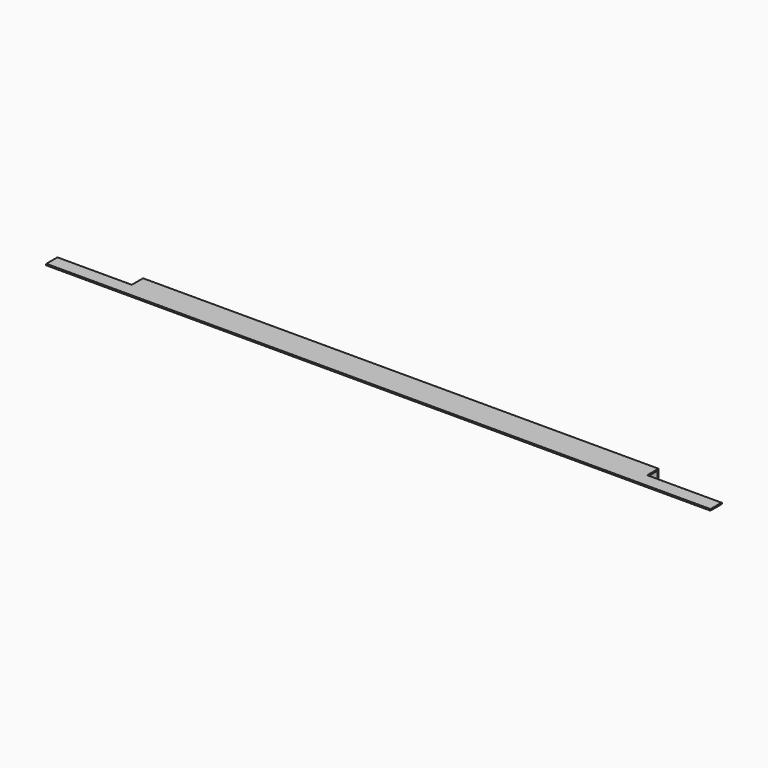
from build123d import *

# Parameters (mm, degrees)
F0_W           = 50.1573085785
F0_H           = 16.5988057852
F1_DEPTH       = 38
F2_DEPTH       = 2
F3_DEPTH       = 894
F4_W           = 19
F4_H           = 2
F5_DEPTH       = 100
F6_W           = 19
F6_H           = 2
F7_DEPTH       = 100
F8_W           = 694
F8_H           = 9.5
F9_DEPTH       = 10
F10_DEPTH      = 7.5
F11_T1_DEPTH   = 21.5048292256
F11_T3_DEPTH   = 101.2524146128
F11_T5_DEPTH   = 17
F11_T7_DEPTH   = 10.9980686292
F11_T9_DEPTH   = 11.2524146128
F11_T11_DEPTH  = 2.7514489274
F11_T13_DEPTH  = 692.9980686292
F11_T15_DEPTH  = 101.2524146128
F11_T17_DEPTH  = 18.4990343146
F11_S21_W      = 0.5515022539
F11_S21_H      = 0.5515022539
F11_T22_DEPTH  = 0.551502254
F11_S27_W      = 0.5515022539
F11_S27_H      = 0.5515022539
F11_T28_DEPTH  = 0.551502254
F11_S33_W      = 0.5515022539
F11_S33_H      = 0.5515022539
F11_T34_DEPTH  = 0.551502254
F11_S39_W      = 0.5515022539
F11_S39_H      = 0.5515022539
F11_T40_DEPTH  = 0.551502254
F11_T47_DEPTH  = 101.2524146128
F11_T51_DEPTH  = 18.2524146128
F11_T58_DEPTH  = 18.2524146128
F11_T62_DEPTH  = 11.2524146128
F11_T69_DEPTH  = 19.7514489274
F11_T73_DEPTH  = 101.2524146128
F11_T80_DEPTH  = 18.2524146128
F11_T84_DEPTH  = 11.2524146128
F11_T91_DEPTH  = 18.2524146128
F11_T95_DEPTH  = 101.2524146128
F11_T102_DEPTH = 19.7514489274
F11_T106_DEPTH = 101.2524146128


# Not quite as in the source:
# - a fillet or chamfer that OpenCascade refuses, or shapes differently, is made with other operations: its cross-section is extruded or revolved along the edge and cut away or added
# - a feature names something its author has since deleted; it is built from what else it names


with BuildPart() as f1:
    # F0 (on Front) → F1 (new body)
    with BuildSketch(Plane.XZ):
        with Locations((-25.0786542892, 8.2994028926)):
            Rectangle(F0_W, F0_H)
    extrude(amount=-F1_DEPTH)

    # F2 (intersect): a face of the model
    f2_faces = [f1.faces().sort_by_distance(p)[0] for p in [
        (-25.0786542892, 19, 0),
    ]]
    extrude(f2_faces, amount=-F2_DEPTH, mode=Mode.INTERSECT)

    # F3 (add): a face of the model
    f3_faces = [f1.faces().sort_by_distance(p)[0] for p in [
        (0, 19, 1),
    ]]
    extrude(f3_faces, amount=-F3_DEPTH)

    # F4 (on face) → F5 (cut)
    with BuildSketch(Plane.YZ):
        with Locations((28.5, 1)):
            Rectangle(F4_W, F4_H)
    extrude(amount=-F5_DEPTH, mode=Mode.SUBTRACT)

    # F6 (on face) → F7 (cut)
    with BuildSketch(Plane(origin=(-894, 0, 0), x_dir=(0, -1, 0), z_dir=(-1, 0, 0))):
        with Locations((-28.5, 1)):
            Rectangle(F6_W, F6_H)
    extrude(amount=-F7_DEPTH, mode=Mode.SUBTRACT)

    # F8 (on face) → F9 (join)
    with BuildSketch(Plane(origin=(0, 0, 0), x_dir=(1, 0, 0), z_dir=(0, 0, -1))):
        with Locations((-447, -33.25)):
            Rectangle(F8_W, F8_H)
    extrude(amount=F9_DEPTH)

    # F10 (cut): a face of the model
    f10_faces = [f1.faces().sort_by_distance(p)[0] for p in [
        (-447, 28.5, -5),
    ]]
    extrude(f10_faces, amount=-F10_DEPTH, mode=Mode.SUBTRACT)

    # F11: fillet of radius 0.5 on 21 edges, made by hand

    # F11_s2 → F11_t1 (cut)
    with BuildSketch(Plane.XZ.offset(-20.2524146128)):
        with BuildLine():
            ThreePointArc((-893.4990343146, -0.0004), (-893.8535533906, 0.1464466094), (-894.0004, 0.5009656854))
            Line((-894.0004, 0.5009656854), (-894.0505365685, 0.5009656854))
            ThreePointArc((-894.0505365685, 0.5009656854), (-894.0501365685, 0.2504828427), (-894.0501365685, 0))
            Line((-894.0501365685, 0), (-894, -0.0501365685))
            ThreePointArc((-894, -0.0501365685), (-893.7495171573, -0.0501365685), (-893.4990343146, -0.0505365685))
            Line((-893.4990343146, -0.0505365685), (-893.4990343146, -0.0004))
        make_face()
        with BuildLine():
            ThreePointArc((0.0004, 0.5009656854), (-0.1464466094, 0.1464466094), (-0.5009656854, -0.0004))
            Line((-0.5009656854, -0.0004), (-0.5009656854, -0.0505365685))
            ThreePointArc((-0.5009656854, -0.0505365685), (-0.2504828427, -0.0501365685), (0, -0.0501365685))
            Line((0, -0.0501365685), (0.0501365685, 0))
            ThreePointArc((0.0501365685, 0), (0.0501365685, 0.2504828427), (0.0505365685, 0.5009656854))
            Line((0.0505365685, 0.5009656854), (0.0004, 0.5009656854))
        make_face()
        with BuildLine():
            ThreePointArc((0.0004, 1.4990343146), (-0.1464466094, 1.8535533906), (-0.5009656854, 2.0004))
            Line((-0.5009656854, 2.0004), (-0.5009656854, 2.0505365685))
            ThreePointArc((-0.5009656854, 2.0505365685), (-0.2504828427, 2.0501365685), (0, 2.0501365685))
            Line((0, 2.0501365685), (0.0501365685, 2))
            ThreePointArc((0.0501365685, 2), (0.0501365685, 1.7495171573), (0.0505365685, 1.4990343146))
            Line((0.0505365685, 1.4990343146), (0.0004, 1.4990343146))
        make_face()
        with BuildLine():
            ThreePointArc((-894.0004, 1.4990343146), (-893.8535533906, 1.8535533906), (-893.4990343146, 2.0004))
            Line((-893.4990343146, 2.0004), (-893.4990343146, 2.0505365685))
            ThreePointArc((-893.4990343146, 2.0505365685), (-893.7495171573, 2.0501365685), (-894, 2.0501365685))
            Line((-894, 2.0501365685), (-894.0501365685, 2))
            ThreePointArc((-894.0501365685, 2), (-894.0501365685, 1.7495171573), (-894.0505365685, 1.4990343146))
            Line((-894.0505365685, 1.4990343146), (-894.0004, 1.4990343146))
        make_face()
    extrude(amount=F11_T1_DEPTH, mode=Mode.SUBTRACT)

    # F11_s4 → F11_t3 (cut)
    with BuildSketch(Plane.YZ.offset(-895.2524146128)):
        with BuildLine():
            ThreePointArc((18.4990343146, -0.0004), (18.8535533906, 0.1464466094), (19.0004, 0.5009656854))
            Line((19.0004, 0.5009656854), (19.0505365685, 0.5009656854))
            ThreePointArc((19.0505365685, 0.5009656854), (19.0501365685, 0.2504828427), (19.0501365685, 0))
            Line((19.0501365685, 0), (19, -0.0501365685))
            ThreePointArc((19, -0.0501365685), (18.7495171573, -0.0501365685), (18.4990343146, -0.0505365685))
            Line((18.4990343146, -0.0505365685), (18.4990343146, -0.0004))
        make_face()
        with BuildLine():
            ThreePointArc((19.0004, 1.4990343146), (18.8535533906, 1.8535533906), (18.4990343146, 2.0004))
            Line((18.4990343146, 2.0004), (18.4990343146, 2.0505365685))
            ThreePointArc((18.4990343146, 2.0505365685), (18.7495171573, 2.0501365685), (19, 2.0501365685))
            Line((19, 2.0501365685), (19.0501365685, 2))
            ThreePointArc((19.0501365685, 2), (19.0501365685, 1.7495171573), (19.0505365685, 1.4990343146))
            Line((19.0505365685, 1.4990343146), (19.0004, 1.4990343146))
        make_face()
    extrude(amount=F11_T3_DEPTH, mode=Mode.SUBTRACT)

    # F11_s6 → F11_t5 (cut)
    with BuildSketch(Plane.XZ.offset(-36)):
        with BuildLine():
            ThreePointArc((-793.4990343146, -0.0004), (-793.8535533906, 0.1464466094), (-794.0004, 0.5009656854))
            Line((-794.0004, 0.5009656854), (-794.0505365685, 0.5009656854))
            ThreePointArc((-794.0505365685, 0.5009656854), (-794.0501365685, 0.2504828427), (-794.0501365685, 0))
            Line((-794.0501365685, 0), (-794, -0.0501365685))
            ThreePointArc((-794, -0.0501365685), (-793.7495171573, -0.0501365685), (-793.4990343146, -0.0505365685))
            Line((-793.4990343146, -0.0505365685), (-793.4990343146, -0.0004))
        make_face()
        with BuildLine():
            ThreePointArc((-100.5009656854, -0.0004), (-100.1464466094, 0.1464466094), (-99.9996, 0.5009656854))
            Line((-99.9996, 0.5009656854), (-99.9494634315, 0.5009656854))
            ThreePointArc((-99.9494634315, 0.5009656854), (-99.9498634315, 0.2504828427), (-99.9498634315, 0))
            Line((-99.9498634315, 0), (-100, -0.0501365685))
            ThreePointArc((-100, -0.0501365685), (-100.2504828427, -0.0501365685), (-100.5009656854, -0.0505365685))
            Line((-100.5009656854, -0.0505365685), (-100.5009656854, -0.0004))
        make_face()
    extrude(amount=F11_T5_DEPTH, mode=Mode.SUBTRACT)

    # F11_s8 → F11_t7 (cut)
    with BuildSketch(Plane.XY.offset(-9.4990343146)):
        with BuildLine():
            ThreePointArc((-793.4990343146, 38.0004), (-793.8535533906, 37.8535533906), (-794.0004, 37.4990343146))
            Line((-794.0004, 37.4990343146), (-794.0505365685, 37.4990343146))
            ThreePointArc((-794.0505365685, 37.4990343146), (-794.0501365685, 37.7495171573), (-794.0501365685, 38))
            Line((-794.0501365685, 38), (-794, 38.0501365685))
            ThreePointArc((-794, 38.0501365685), (-793.7495171573, 38.0501365685), (-793.4990343146, 38.0505365685))
            Line((-793.4990343146, 38.0505365685), (-793.4990343146, 38.0004))
        make_face()
        with BuildLine():
            ThreePointArc((-99.9996, 37.4990343146), (-100.1464466094, 37.8535533906), (-100.5009656854, 38.0004))
            Line((-100.5009656854, 38.0004), (-100.5009656854, 38.0505365685))
            ThreePointArc((-100.5009656854, 38.0505365685), (-100.2504828427, 38.0501365685), (-100, 38.0501365685))
            Line((-100, 38.0501365685), (-99.9498634315, 38))
            ThreePointArc((-99.9498634315, 38), (-99.9498634315, 37.7495171573), (-99.9494634315, 37.4990343146))
            Line((-99.9494634315, 37.4990343146), (-99.9996, 37.4990343146))
        make_face()
    extrude(amount=F11_T7_DEPTH, mode=Mode.SUBTRACT)

    # F11_s10 → F11_t9 (cut)
    with BuildSketch(Plane.XY.offset(-11.2524146128)):
        with BuildLine():
            ThreePointArc((-793.4990343146, 35.9996), (-793.8535533906, 36.1464466094), (-794.0004, 36.5009656854))
            Line((-794.0004, 36.5009656854), (-794.0505365685, 36.5009656854))
            ThreePointArc((-794.0505365685, 36.5009656854), (-794.0501365685, 36.2504828427), (-794.0501365685, 36))
            Line((-794.0501365685, 36), (-794, 35.9498634315))
            ThreePointArc((-794, 35.9498634315), (-793.7495171573, 35.9498634315), (-793.4990343146, 35.9494634315))
            Line((-793.4990343146, 35.9494634315), (-793.4990343146, 35.9996))
        make_face()
        with BuildLine():
            ThreePointArc((-99.9996, 36.5009656854), (-100.1464466094, 36.1464466094), (-100.5009656854, 35.9996))
            Line((-100.5009656854, 35.9996), (-100.5009656854, 35.9494634315))
            ThreePointArc((-100.5009656854, 35.9494634315), (-100.2504828427, 35.9498634315), (-100, 35.9498634315))
            Line((-100, 35.9498634315), (-99.9498634315, 36))
            ThreePointArc((-99.9498634315, 36), (-99.9498634315, 36.2504828427), (-99.9494634315, 36.5009656854))
            Line((-99.9494634315, 36.5009656854), (-99.9996, 36.5009656854))
        make_face()
    extrude(amount=F11_T9_DEPTH, mode=Mode.SUBTRACT)

    # F11_s12 → F11_t11 (cut)
    with BuildSketch(Plane.XZ.offset(-37.4990343146)):
        with BuildLine():
            ThreePointArc((-793.4990343146, -10.0004), (-793.8535533906, -9.8535533906), (-794.0004, -9.4990343146))
            Line((-794.0004, -9.4990343146), (-794.0505365685, -9.4990343146))
            ThreePointArc((-794.0505365685, -9.4990343146), (-794.0501365685, -9.7495171573), (-794.0501365685, -10))
            Line((-794.0501365685, -10), (-794, -10.0501365685))
            ThreePointArc((-794, -10.0501365685), (-793.7495171573, -10.0501365685), (-793.4990343146, -10.0505365685))
            Line((-793.4990343146, -10.0505365685), (-793.4990343146, -10.0004))
        make_face()
        with BuildLine():
            ThreePointArc((-99.9996, -9.4990343146), (-100.1464466094, -9.8535533906), (-100.5009656854, -10.0004))
            Line((-100.5009656854, -10.0004), (-100.5009656854, -10.0505365685))
            ThreePointArc((-100.5009656854, -10.0505365685), (-100.2504828427, -10.0501365685), (-100, -10.0501365685))
            Line((-100, -10.0501365685), (-99.9498634315, -10))
            ThreePointArc((-99.9498634315, -10), (-99.9498634315, -9.7495171573), (-99.9494634315, -9.4990343146))
            Line((-99.9494634315, -9.4990343146), (-99.9996, -9.4990343146))
        make_face()
    extrude(amount=F11_T11_DEPTH, mode=Mode.SUBTRACT)

    # F11_s14 → F11_t13 (cut)
    with BuildSketch(Plane.YZ.offset(-793.4990343146)):
        with BuildLine():
            ThreePointArc((37.4990343146, -10.0004), (37.8535533906, -9.8535533906), (38.0004, -9.4990343146))
            Line((38.0004, -9.4990343146), (38.0505365685, -9.4990343146))
            ThreePointArc((38.0505365685, -9.4990343146), (38.0501365685, -9.7495171573), (38.0501365685, -10))
            Line((38.0501365685, -10), (38, -10.0501365685))
            ThreePointArc((38, -10.0501365685), (37.7495171573, -10.0501365685), (37.4990343146, -10.0505365685))
            Line((37.4990343146, -10.0505365685), (37.4990343146, -10.0004))
        make_face()
        with BuildLine():
            ThreePointArc((38.0004, 1.4990343146), (37.8535533906, 1.8535533906), (37.4990343146, 2.0004))
            Line((37.4990343146, 2.0004), (37.4990343146, 2.0505365685))
            ThreePointArc((37.4990343146, 2.0505365685), (37.7495171573, 2.0501365685), (38, 2.0501365685))
            Line((38, 2.0501365685), (38.0501365685, 2))
            ThreePointArc((38.0501365685, 2), (38.0501365685, 1.7495171573), (38.0505365685, 1.4990343146))
            Line((38.0505365685, 1.4990343146), (38.0004, 1.4990343146))
        make_face()
    extrude(amount=F11_T13_DEPTH, mode=Mode.SUBTRACT)

    # F11_s16 → F11_t15 (cut)
    with BuildSketch(Plane.YZ.offset(-100)):
        with BuildLine():
            ThreePointArc((19.0004, 1.4990343146), (18.8535533906, 1.8535533906), (18.4990343146, 2.0004))
            Line((18.4990343146, 2.0004), (18.4990343146, 2.0505365685))
            ThreePointArc((18.4990343146, 2.0505365685), (18.7495171573, 2.0501365685), (19, 2.0501365685))
            Line((19, 2.0501365685), (19.0501365685, 2))
            ThreePointArc((19.0501365685, 2), (19.0501365685, 1.7495171573), (19.0505365685, 1.4990343146))
            Line((19.0505365685, 1.4990343146), (19.0004, 1.4990343146))
        make_face()
        with BuildLine():
            ThreePointArc((18.4990343146, -0.0004), (18.8535533906, 0.1464466094), (19.0004, 0.5009656854))
            Line((19.0004, 0.5009656854), (19.0505365685, 0.5009656854))
            ThreePointArc((19.0505365685, 0.5009656854), (19.0501365685, 0.2504828427), (19.0501365685, 0))
            Line((19.0501365685, 0), (19, -0.0501365685))
            ThreePointArc((19, -0.0501365685), (18.7495171573, -0.0501365685), (18.4990343146, -0.0505365685))
            Line((18.4990343146, -0.0505365685), (18.4990343146, -0.0004))
        make_face()
    extrude(amount=F11_T15_DEPTH, mode=Mode.SUBTRACT)

    # F11_s18 → F11_t17 (cut)
    with BuildSketch(Plane.XZ.offset(-37.4990343146)):
        with BuildLine():
            ThreePointArc((-99.9996, 1.4990343146), (-100.1464466094, 1.8535533906), (-100.5009656854, 2.0004))
            Line((-100.5009656854, 2.0004), (-100.5009656854, 2.0505365685))
            ThreePointArc((-100.5009656854, 2.0505365685), (-100.2504828427, 2.0501365685), (-100, 2.0501365685))
            Line((-100, 2.0501365685), (-99.9498634315, 2))
            ThreePointArc((-99.9498634315, 2), (-99.9498634315, 1.7495171573), (-99.9494634315, 1.4990343146))
            Line((-99.9494634315, 1.4990343146), (-99.9996, 1.4990343146))
        make_face()
        with BuildLine():
            ThreePointArc((-794.0004, 1.4990343146), (-793.8535533906, 1.8535533906), (-793.4990343146, 2.0004))
            Line((-793.4990343146, 2.0004), (-793.4990343146, 2.0505365685))
            ThreePointArc((-793.4990343146, 2.0505365685), (-793.7495171573, 2.0501365685), (-794, 2.0501365685))
            Line((-794, 2.0501365685), (-794.0501365685, 2))
            ThreePointArc((-794.0501365685, 2), (-794.0501365685, 1.7495171573), (-794.0505365685, 1.4990343146))
            Line((-794.0505365685, 1.4990343146), (-794.0004, 1.4990343146))
        make_face()
    extrude(amount=F11_T17_DEPTH, mode=Mode.SUBTRACT)


with BuildPart() as f11_tool20:
    # F11_s21 → F11_t22 (new body)
    with BuildSketch(Plane.XY.offset(-9.4990343146)):
        with Locations((-793.7747854415, 37.7747854416)):
            Rectangle(F11_S21_W, F11_S21_H)
    extrude(amount=-F11_T22_DEPTH)

    # F11_s23 → F11_t24 (revolve, cut)
    with BuildSketch(Plane(origin=(-793.4990343146, 37.4990343146, -9.4990343146), x_dir=(0.7071067812, -0.7071067812, 0), z_dir=(0.7071067812, 0.7071067812, 0))):
        with BuildLine():
            ThreePointArc((0, -0.5013656854), (0.5013656854, 0), (0, 0.5013656854))
            Line((0, 0.5013656854), (0, -0.5013656854))
        make_face()
    revolve(axis=Axis((-793.4990343146, 37.4990343146, -9.4990343146), (0, 0, -1)), mode=Mode.SUBTRACT)


with BuildPart() as f1_1:
    add(f1.part)

    # F11_t19: cut F11_tool20
    add(f11_tool20.part, mode=Mode.SUBTRACT)


with BuildPart() as f11_tool26:
    # F11_s27 → F11_t28 (new body)
    with BuildSketch(Plane.XY.offset(1.4990343146)):
        with Locations((-793.7747854415, 37.7747854416)):
            Rectangle(F11_S27_W, F11_S27_H)
    extrude(amount=F11_T28_DEPTH)

    # F11_s29 → F11_t30 (revolve, cut)
    with BuildSketch(Plane(origin=(-793.4990343146, 37.4990343146, 1.4990343146), x_dir=(0.7071067812, -0.7071067812, 0), z_dir=(-0.7071067812, -0.7071067812, 0))):
        with BuildLine():
            ThreePointArc((0, -0.5013656854), (0.5013656854, 0), (0, 0.5013656854))
            Line((0, 0.5013656854), (0, -0.5013656854))
        make_face()
    revolve(axis=Axis((-793.4990343146, 37.4990343146, 1.4990343146), (0, 0, 1)), mode=Mode.SUBTRACT)


with BuildPart() as f1_2:
    add(f1_1.part)

    # F11_t25: cut F11_tool26
    add(f11_tool26.part, mode=Mode.SUBTRACT)


with BuildPart() as f11_tool32:
    # F11_s33 → F11_t34 (new body)
    with BuildSketch(Plane.YZ.offset(-100.5009656854)):
        with Locations((37.7747854416, -9.7747854415)):
            Rectangle(F11_S33_W, F11_S33_H)
    extrude(amount=F11_T34_DEPTH)

    # F11_s35 → F11_t36 (revolve, cut)
    with BuildSketch(Plane(origin=(-100.5009656854, 37.4990343146, -9.4990343146), x_dir=(0, -0.7071067812, 0.7071067812), z_dir=(0, 0.7071067812, 0.7071067812))):
        with BuildLine():
            ThreePointArc((0, -0.5013656854), (0.5013656854, 0), (0, 0.5013656854))
            Line((0, 0.5013656854), (0, -0.5013656854))
        make_face()
    revolve(axis=Axis((-100.5009656854, 37.4990343146, -9.4990343146), (1, 0, 0)), mode=Mode.SUBTRACT)


with BuildPart() as f1_3:
    add(f1_2.part)

    # F11_t31: cut F11_tool32
    add(f11_tool32.part, mode=Mode.SUBTRACT)


with BuildPart() as f11_tool38:
    # F11_s39 → F11_t40 (new body)
    with BuildSketch(Plane.YZ.offset(-100.5009656854)):
        with Locations((37.7747854416, 1.7747854416)):
            Rectangle(F11_S39_W, F11_S39_H)
    extrude(amount=F11_T40_DEPTH)

    # F11_s41 → F11_t42 (revolve, cut)
    with BuildSketch(Plane(origin=(-100.5009656854, 37.4990343146, 1.4990343146), x_dir=(0, -0.7071067812, -0.7071067812), z_dir=(0, -0.7071067812, 0.7071067812))):
        with BuildLine():
            ThreePointArc((0, -0.5013656854), (0.5013656854, 0), (0, 0.5013656854))
            Line((0, 0.5013656854), (0, -0.5013656854))
        make_face()
    revolve(axis=Axis((-100.5009656854, 37.4990343146, 1.4990343146), (1, 0, 0)), mode=Mode.SUBTRACT)


with BuildPart() as f1_4:
    add(f1_3.part)

    # F11_t37: cut F11_tool38
    add(f11_tool38.part, mode=Mode.SUBTRACT)


with BuildPart() as f11_tool45:
    # F11_s46 → F11_t47 (new body)
    with BuildSketch(Plane.YZ.offset(-894)):
        with BuildLine():
            ThreePointArc((18.4990343146, -0.0004), (18.8535533906, 0.1464466094), (19.0004, 0.5009656854))
            Line((19.0004, 0.5009656854), (19.0505365685, 0.5009656854))
            ThreePointArc((19.0505365685, 0.5009656854), (19.0501365685, 0.2504828427), (19.0501365685, 0))
            Line((19.0501365685, 0), (19, -0.0501365685))
            ThreePointArc((19, -0.0501365685), (18.7495171573, -0.0501365685), (18.4990343146, -0.0505365685))
            Line((18.4990343146, -0.0505365685), (18.4990343146, -0.0004))
        make_face()
    extrude(amount=F11_T47_DEPTH)

    split(bisect_by=Plane.YZ.offset(-794), keep=Keep.TOP)


with BuildPart() as f11_tool49:
    # F11_s50 → F11_t51 (new body)
    with BuildSketch(Plane.XZ.offset(-17.7475853872)):
        with BuildLine():
            ThreePointArc((-793.4990343146, -0.0004), (-793.8535533906, 0.1464466094), (-794.0004, 0.5009656854))
            Line((-794.0004, 0.5009656854), (-794.0505365685, 0.5009656854))
            ThreePointArc((-794.0505365685, 0.5009656854), (-794.0501365685, 0.2504828427), (-794.0501365685, 0))
            Line((-794.0501365685, 0), (-794, -0.0501365685))
            ThreePointArc((-794, -0.0501365685), (-793.7495171573, -0.0501365685), (-793.4990343146, -0.0505365685))
            Line((-793.4990343146, -0.0505365685), (-793.4990343146, -0.0004))
        make_face()
    extrude(amount=-F11_T51_DEPTH)

    split(bisect_by=Plane.XZ.offset(-19), keep=Keep.TOP)


with BuildPart() as f11_tool45_1:
    add(f11_tool45.part)

    # F11_t53: intersect F11_tool49
    add(f11_tool49.part, mode=Mode.INTERSECT)


with BuildPart() as f1_5:
    add(f1_4.part)

    # F11_t43: cut F11_tool45
    add(f11_tool45_1.part, mode=Mode.SUBTRACT)


with BuildPart() as f11_tool56:
    # F11_s57 → F11_t58 (new body)
    with BuildSketch(Plane.XZ.offset(-19)):
        with BuildLine():
            ThreePointArc((-793.4990343146, -0.0004), (-793.8535533906, 0.1464466094), (-794.0004, 0.5009656854))
            Line((-794.0004, 0.5009656854), (-794.0505365685, 0.5009656854))
            ThreePointArc((-794.0505365685, 0.5009656854), (-794.0501365685, 0.2504828427), (-794.0501365685, 0))
            Line((-794.0501365685, 0), (-794, -0.0501365685))
            ThreePointArc((-794, -0.0501365685), (-793.7495171573, -0.0501365685), (-793.4990343146, -0.0505365685))
            Line((-793.4990343146, -0.0505365685), (-793.4990343146, -0.0004))
        make_face()
    extrude(amount=-F11_T58_DEPTH)

    split(bisect_by=Plane.XZ.offset(-36), keep=Keep.BOTTOM)


with BuildPart() as f11_tool60:
    # F11_s61 → F11_t62 (new body)
    with BuildSketch(Plane.XY.offset(1.2524146128)):
        with BuildLine():
            ThreePointArc((-793.4990343146, 35.9996), (-793.8535533906, 36.1464466094), (-794.0004, 36.5009656854))
            Line((-794.0004, 36.5009656854), (-794.0505365685, 36.5009656854))
            ThreePointArc((-794.0505365685, 36.5009656854), (-794.0501365685, 36.2504828427), (-794.0501365685, 36))
            Line((-794.0501365685, 36), (-794, 35.9498634315))
            ThreePointArc((-794, 35.9498634315), (-793.7495171573, 35.9498634315), (-793.4990343146, 35.9494634315))
            Line((-793.4990343146, 35.9494634315), (-793.4990343146, 35.9996))
        make_face()
    extrude(amount=-F11_T62_DEPTH)

    split(bisect_by=Plane.XY, keep=Keep.TOP)


with BuildPart() as f11_tool56_1:
    add(f11_tool56.part)

    # F11_t64: intersect F11_tool60
    add(f11_tool60.part, mode=Mode.INTERSECT)


with BuildPart() as f1_6:
    add(f1_5.part)

    # F11_t54: cut F11_tool56
    add(f11_tool56_1.part, mode=Mode.SUBTRACT)


with BuildPart() as f11_tool67:
    # F11_s68 → F11_t69 (new body)
    with BuildSketch(Plane.XZ.offset(-37.4990343146)):
        with BuildLine():
            ThreePointArc((-99.9996, 1.4990343146), (-100.1464466094, 1.8535533906), (-100.5009656854, 2.0004))
            Line((-100.5009656854, 2.0004), (-100.5009656854, 2.0505365685))
            ThreePointArc((-100.5009656854, 2.0505365685), (-100.2504828427, 2.0501365685), (-100, 2.0501365685))
            Line((-100, 2.0501365685), (-99.9498634315, 2))
            ThreePointArc((-99.9498634315, 2), (-99.9498634315, 1.7495171573), (-99.9494634315, 1.4990343146))
            Line((-99.9494634315, 1.4990343146), (-99.9996, 1.4990343146))
        make_face()
    extrude(amount=F11_T69_DEPTH)

    split(bisect_by=Plane.XZ.offset(-19), keep=Keep.TOP)


with BuildPart() as f11_tool71:
    # F11_s72 → F11_t73 (new body)
    with BuildSketch(Plane.YZ):
        with BuildLine():
            ThreePointArc((19.0004, 1.4990343146), (18.8535533906, 1.8535533906), (18.4990343146, 2.0004))
            Line((18.4990343146, 2.0004), (18.4990343146, 2.0505365685))
            ThreePointArc((18.4990343146, 2.0505365685), (18.7495171573, 2.0501365685), (19, 2.0501365685))
            Line((19, 2.0501365685), (19.0501365685, 2))
            ThreePointArc((19.0501365685, 2), (19.0501365685, 1.7495171573), (19.0505365685, 1.4990343146))
            Line((19.0505365685, 1.4990343146), (19.0004, 1.4990343146))
        make_face()
    extrude(amount=-F11_T73_DEPTH)

    split(bisect_by=Plane.YZ.offset(-100), keep=Keep.BOTTOM)


with BuildPart() as f11_tool67_1:
    add(f11_tool67.part)

    # F11_t75: intersect F11_tool71
    add(f11_tool71.part, mode=Mode.INTERSECT)


with BuildPart() as f1_7:
    add(f1_6.part)

    # F11_t65: cut F11_tool67
    add(f11_tool67_1.part, mode=Mode.SUBTRACT)


with BuildPart() as f11_tool78:
    # F11_s79 → F11_t80 (new body)
    with BuildSketch(Plane.XZ.offset(-37.2524146128)):
        with BuildLine():
            ThreePointArc((-100.5009656854, -0.0004), (-100.1464466094, 0.1464466094), (-99.9996, 0.5009656854))
            Line((-99.9996, 0.5009656854), (-99.9494634315, 0.5009656854))
            ThreePointArc((-99.9494634315, 0.5009656854), (-99.9498634315, 0.2504828427), (-99.9498634315, 0))
            Line((-99.9498634315, 0), (-100, -0.0501365685))
            ThreePointArc((-100, -0.0501365685), (-100.2504828427, -0.0501365685), (-100.5009656854, -0.0505365685))
            Line((-100.5009656854, -0.0505365685), (-100.5009656854, -0.0004))
        make_face()
    extrude(amount=F11_T80_DEPTH)

    split(bisect_by=Plane.XZ.offset(-36), keep=Keep.BOTTOM)


with BuildPart() as f11_tool82:
    # F11_s83 → F11_t84 (new body)
    with BuildSketch(Plane.XY.offset(1.2524146128)):
        with BuildLine():
            ThreePointArc((-99.9996, 36.5009656854), (-100.1464466094, 36.1464466094), (-100.5009656854, 35.9996))
            Line((-100.5009656854, 35.9996), (-100.5009656854, 35.9494634315))
            ThreePointArc((-100.5009656854, 35.9494634315), (-100.2504828427, 35.9498634315), (-100, 35.9498634315))
            Line((-100, 35.9498634315), (-99.9498634315, 36))
            ThreePointArc((-99.9498634315, 36), (-99.9498634315, 36.2504828427), (-99.9494634315, 36.5009656854))
            Line((-99.9494634315, 36.5009656854), (-99.9996, 36.5009656854))
        make_face()
    extrude(amount=-F11_T84_DEPTH)

    split(bisect_by=Plane.XY, keep=Keep.TOP)


with BuildPart() as f11_tool78_1:
    add(f11_tool78.part)

    # F11_t86: intersect F11_tool82
    add(f11_tool82.part, mode=Mode.INTERSECT)


with BuildPart() as f1_8:
    add(f1_7.part)

    # F11_t76: cut F11_tool78
    add(f11_tool78_1.part, mode=Mode.SUBTRACT)


with BuildPart() as f11_tool89:
    # F11_s90 → F11_t91 (new body)
    with BuildSketch(Plane.XZ.offset(-36)):
        with BuildLine():
            ThreePointArc((-100.5009656854, -0.0004), (-100.1464466094, 0.1464466094), (-99.9996, 0.5009656854))
            Line((-99.9996, 0.5009656854), (-99.9494634315, 0.5009656854))
            ThreePointArc((-99.9494634315, 0.5009656854), (-99.9498634315, 0.2504828427), (-99.9498634315, 0))
            Line((-99.9498634315, 0), (-100, -0.0501365685))
            ThreePointArc((-100, -0.0501365685), (-100.2504828427, -0.0501365685), (-100.5009656854, -0.0505365685))
            Line((-100.5009656854, -0.0505365685), (-100.5009656854, -0.0004))
        make_face()
    extrude(amount=F11_T91_DEPTH)

    split(bisect_by=Plane.XZ.offset(-19), keep=Keep.TOP)


with BuildPart() as f11_tool93:
    # F11_s94 → F11_t95 (new body)
    with BuildSketch(Plane.YZ):
        with BuildLine():
            ThreePointArc((18.4990343146, -0.0004), (18.8535533906, 0.1464466094), (19.0004, 0.5009656854))
            Line((19.0004, 0.5009656854), (19.0505365685, 0.5009656854))
            ThreePointArc((19.0505365685, 0.5009656854), (19.0501365685, 0.2504828427), (19.0501365685, 0))
            Line((19.0501365685, 0), (19, -0.0501365685))
            ThreePointArc((19, -0.0501365685), (18.7495171573, -0.0501365685), (18.4990343146, -0.0505365685))
            Line((18.4990343146, -0.0505365685), (18.4990343146, -0.0004))
        make_face()
    extrude(amount=-F11_T95_DEPTH)

    split(bisect_by=Plane.YZ.offset(-100), keep=Keep.BOTTOM)


with BuildPart() as f11_tool89_1:
    add(f11_tool89.part)

    # F11_t97: intersect F11_tool93
    add(f11_tool93.part, mode=Mode.INTERSECT)


with BuildPart() as f1_9:
    add(f1_8.part)

    # F11_t87: cut F11_tool89
    add(f11_tool89_1.part, mode=Mode.SUBTRACT)


with BuildPart() as f11_tool100:
    # F11_s101 → F11_t102 (new body)
    with BuildSketch(Plane.XZ.offset(-17.7475853872)):
        with BuildLine():
            ThreePointArc((-794.0004, 1.4990343146), (-793.8535533906, 1.8535533906), (-793.4990343146, 2.0004))
            Line((-793.4990343146, 2.0004), (-793.4990343146, 2.0505365685))
            ThreePointArc((-793.4990343146, 2.0505365685), (-793.7495171573, 2.0501365685), (-794, 2.0501365685))
            Line((-794, 2.0501365685), (-794.0501365685, 2))
            ThreePointArc((-794.0501365685, 2), (-794.0501365685, 1.7495171573), (-794.0505365685, 1.4990343146))
            Line((-794.0505365685, 1.4990343146), (-794.0004, 1.4990343146))
        make_face()
    extrude(amount=-F11_T102_DEPTH)

    split(bisect_by=Plane.XZ.offset(-19), keep=Keep.TOP)


with BuildPart() as f11_tool104:
    # F11_s105 → F11_t106 (new body)
    with BuildSketch(Plane.YZ.offset(-894)):
        with BuildLine():
            ThreePointArc((19.0004, 1.4990343146), (18.8535533906, 1.8535533906), (18.4990343146, 2.0004))
            Line((18.4990343146, 2.0004), (18.4990343146, 2.0505365685))
            ThreePointArc((18.4990343146, 2.0505365685), (18.7495171573, 2.0501365685), (19, 2.0501365685))
            Line((19, 2.0501365685), (19.0501365685, 2))
            ThreePointArc((19.0501365685, 2), (19.0501365685, 1.7495171573), (19.0505365685, 1.4990343146))
            Line((19.0505365685, 1.4990343146), (19.0004, 1.4990343146))
        make_face()
    extrude(amount=F11_T106_DEPTH)

    split(bisect_by=Plane.YZ.offset(-794), keep=Keep.TOP)


with BuildPart() as f11_tool100_1:
    add(f11_tool100.part)

    # F11_t108: intersect F11_tool104
    add(f11_tool104.part, mode=Mode.INTERSECT)


with BuildPart() as f1_10:
    add(f1_9.part)

    # F11_t98: cut F11_tool100
    add(f11_tool100_1.part, mode=Mode.SUBTRACT)


solid = f1_10.part
